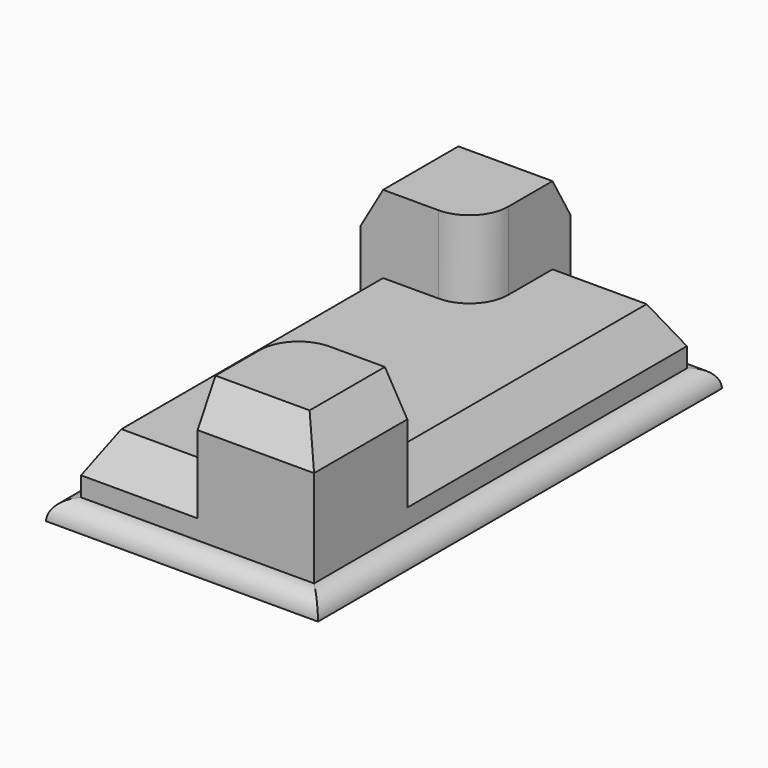
from build123d import *

# Parameters (mm, degrees)
F0_W        = 88.9000007987
F0_H        = 165.1000007987
F1_DEPTH    = 6.35
F2_DEPTH    = 25.4
F3_DEPTH    = 50.8
F4_C1_SIZE2 = 7.3323484187
F4_C1_SIZE  = 12.7
F4_C2_SIZE2 = 7.3323484187
F4_C2_SIZE  = 12.7
F4_C3_SIZE2 = 7.3323484187
F4_C3_SIZE  = 12.7
F4_C4_SIZE2 = 12.7
F4_C4_SIZE  = 7.3323484187
F4_C5_SIZE2 = 7.3323484187
F4_C5_SIZE  = 12.7
F5_C1_SIZE2 = 12.7
F5_C1_SIZE  = 7.3323484187
F5_C2_SIZE2 = 12.7
F5_C2_SIZE  = 7.3323484187
F5_C3_SIZE2 = 7.3323484187
F5_C3_SIZE  = 12.7
F6_R        = 6.34999


# Not quite as in the source:
# - a fillet or chamfer is up to 0.001 mm smaller than in the source, because OpenCascade refuses the exact size


with BuildPart() as f1:
    # F0 (on Top) → F1 (new body)
    with BuildSketch(Plane.XY):
        Rectangle(F0_W, F0_H)
        Polygon((-38.1, 38.1), (-38.1, 76.2), (0, 76.2), (38.1, 76.2), (38.1, -38.1), (38.1, -76.2), (0, -76.2), (-38.1, -76.2), align=None, mode=Mode.SUBTRACT)
    extrude(amount=F1_DEPTH)

    # F0 (on Top) → F2 (join)
    with BuildSketch(Plane.XY):
        with BuildLine():
            Line((38.1, 76.2), (0, 76.2))
            Line((0, 76.2), (0, 50.8))
            ThreePointArc((0, 50.8), (-3.7197438789, 41.8197438789), (-12.7, 38.1))
            Line((-12.7, 38.1), (-38.1, 38.1))
            Line((-38.1, 38.1), (-38.1, -76.2))
            Line((-38.1, -76.2), (0, -76.2))
            Line((0, -76.2), (0, -50.8))
            ThreePointArc((0, -50.8), (3.7197438789, -41.8197438789), (12.7, -38.1))
            Line((12.7, -38.1), (38.1, -38.1))
            Line((38.1, -38.1), (38.1, 76.2))
        make_face()
    extrude(amount=F2_DEPTH)

    # F0 (on Top) → F3 (join)
    with BuildSketch(Plane.XY):
        with BuildLine():
            Line((0, 76.2), (-38.1, 76.2))
            Line((-38.1, 76.2), (-38.1, 38.1))
            Line((-38.1, 38.1), (-12.7, 38.1))
            ThreePointArc((-12.7, 38.1), (-3.7197438789, 41.8197438789), (0, 50.8))
            Line((0, 50.8), (0, 76.2))
        make_face()
        with BuildLine():
            Line((38.1, -76.2), (38.1, -38.1))
            Line((38.1, -38.1), (12.7, -38.1))
            ThreePointArc((12.7, -38.1), (3.7197438789, -41.8197438789), (0, -50.8))
            Line((0, -50.8), (0, -76.2))
            Line((0, -76.2), (38.1, -76.2))
        make_face()
    extrude(amount=F3_DEPTH)

    # F4: chamfer of 12.7 x 7.3323484187 on 5 edges, made by hand

    # F4_c1
    f4_c1_edges = [f1.edges().sort_by_distance(p)[0] for p in [
        (-19.05, -76.2, 25.4),
    ]]
    f4_c1_side = f1.faces().sort_by_distance((-19.05, -76.2, 25.2533530316))[0]
    chamfer(f4_c1_edges, length=F4_C1_SIZE, length2=F4_C1_SIZE2, reference=f4_c1_side)

    # F4_c2
    f4_c2_edges = [f1.edges().sort_by_distance(p)[0] for p in [
        (19.05, -76.2, 50.8),
    ]]
    f4_c2_side = f1.faces().sort_by_distance((19.05, -76.2, 50.6533530316))[0]
    chamfer(f4_c2_edges, length=F4_C2_SIZE, length2=F4_C2_SIZE2, reference=f4_c2_side)

    # F4_c3
    f4_c3_edges = [f1.edges().sort_by_distance(p)[0] for p in [
        (38.1, -53.4838257906, 50.8),
    ]]
    f4_c3_side = f1.faces().sort_by_distance((38.1, -53.4838257906, 50.6533530316))[0]
    chamfer(f4_c3_edges, length=F4_C3_SIZE, length2=F4_C3_SIZE2, reference=f4_c3_side)

    # F4_c4
    f4_c4_edges = [f1.edges().sort_by_distance(p)[0] for p in [
        (-38.1, -15.3838257906, 25.4),
    ]]
    f4_c4_side = f1.faces().sort_by_distance((-37.9533530316, -15.3838257906, 25.4))[0]
    chamfer(f4_c4_edges, length=F4_C4_SIZE, length2=F4_C4_SIZE2, reference=f4_c4_side)

    # F4_c5
    f4_c5_edges = [f1.edges().sort_by_distance(p)[0] for p in [
        (-38.1, 57.15, 50.8),
    ]]
    f4_c5_side = f1.faces().sort_by_distance((-38.1, 57.15, 50.6533530316))[0]
    chamfer(f4_c5_edges, length=F4_C5_SIZE, length2=F4_C5_SIZE2, reference=f4_c5_side)

    # F5: chamfer of 12.7 x 7.3323484187 on 3 edges, made by hand

    # F5_c1
    f5_c1_edges = [f1.edges().sort_by_distance(p)[0] for p in [
        (-15.3838257906, 76.2, 50.8),
    ]]
    f5_c1_side = f1.faces().sort_by_distance((-15.3838257906, 76.0533530316, 50.8))[0]
    chamfer(f5_c1_edges, length=F5_C1_SIZE, length2=F5_C1_SIZE2, reference=f5_c1_side)

    # F5_c2
    f5_c2_edges = [f1.edges().sort_by_distance(p)[0] for p in [
        (38.1, 19.05, 25.4),
    ]]
    f5_c2_side = f1.faces().sort_by_distance((37.9533530316, 19.05, 25.4))[0]
    chamfer(f5_c2_edges, length=F5_C2_SIZE, length2=F5_C2_SIZE2, reference=f5_c2_side)

    # F5_c3
    f5_c3_edges = [f1.edges().sort_by_distance(p)[0] for p in [
        (15.3838257906, 76.2, 25.4),
    ]]
    f5_c3_side = f1.faces().sort_by_distance((15.3838257906, 76.2, 25.2533530316))[0]
    chamfer(f5_c3_edges, length=F5_C3_SIZE, length2=F5_C3_SIZE2, reference=f5_c3_side)

    # F6 (radius 6.35 in the source; OpenCascade refuses exactly that, so slightly less here)
    f6_edges = [f1.edges().sort_by_distance(p)[0] for p in [
        (44.45, 0, 6.35),
        (0, -82.55, 6.35),
        (-44.45, 0, 6.35),
        (0, 82.55, 6.35),
    ]]
    fillet(f6_edges, radius=F6_R)


solid = f1.part
